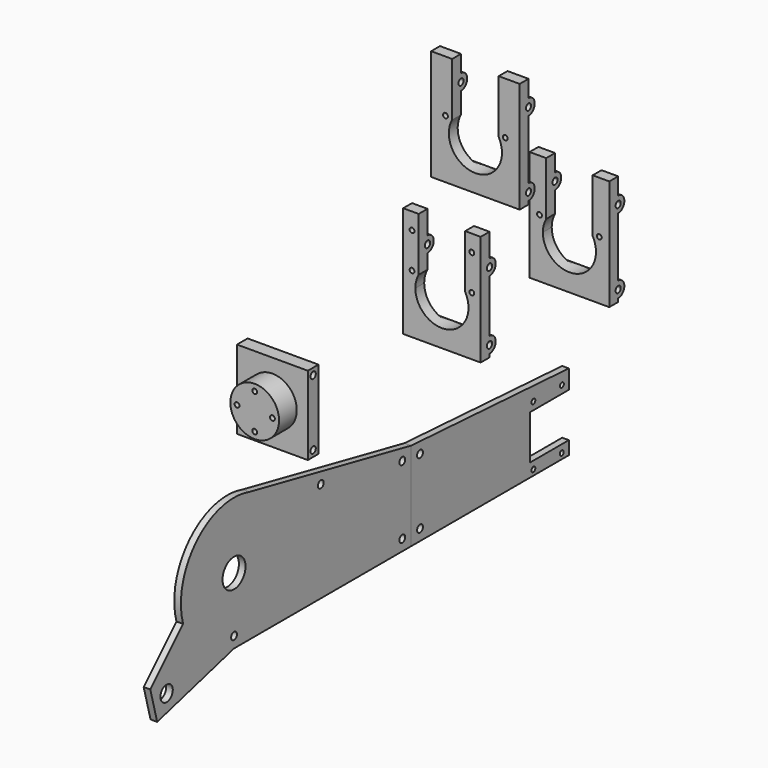
from build123d import *

# Parameters (mm, degrees)
F0_R            = 1.65
F0_R_2          = 1.1
F1_DEPTH        = 3
F2_R            = 3.5
F2_R_2          = 1.65
F2_R_3          = 6.5
F3_DEPTH        = 3
F5_DEPTH        = 35
F7_D            = 2.2
F7_DEPTH        = 12
F7_CBORE_D      = 4
F7_CBORE_DEPTH  = 2
F7_TIP          = 0.6609466809
F6_W            = 21
F6_H            = 10.579
F8_DEPTH        = 25
F8_DEPTH_BACK   = 25
F9_W            = 6
F9_H            = 35.53
F10_DEPTH       = 32
F11_D           = 3
F12_R           = 11
F13_DEPTH       = 16
F14_D           = 2.2
F14_CBORE_D     = 4
F14_CBORE_DEPTH = 13
F16_DEPTH       = 36
F17_W           = 21
F17_H           = 7.7
F18_DEPTH       = 222.8771624415
F18_DEPTH_BACK  = 25
F19_D           = 2.2
F19_DEPTH       = 12
F19_CBORE_D     = 4
F19_CBORE_DEPTH = 2
F19_TIP         = 0.6609466809
F21_DEPTH       = 40
F22_W           = 21
F22_H           = 7.7
F23_DEPTH       = 12.5
F24_D           = 2.2
F24_CBORE_D     = 4
F24_CBORE_DEPTH = 2


# Not quite as in the source:
# - a feature names something its author has since deleted; it is built from what else it names


with BuildPart() as f1:
    # F0 (on Right) → F1 (new body)
    with BuildSketch(Plane.YZ):
        Polygon((134.868821919, -66.8961822494), (45.859821919, -61.4187053263), (45.859821919, -101.4187053263), (134.868821919, -101.4187053263), (134.868821919, -95.4187053263), (112.868821919, -95.4187053263), (112.868821919, -75.4187053263), (134.868821919, -75.4187053263), align=None)
        with Locations((50.859821919, -96.4187053263)):
            Circle(F0_R, mode=Mode.SUBTRACT)
        with Locations((114.868821919, -98.9187053263)):
            Circle(F0_R_2, mode=Mode.SUBTRACT)
        with Locations((130.868821919, -98.9187053263)):
            Circle(F0_R_2, mode=Mode.SUBTRACT)
        with Locations((50.859821919, -66.7358561433)):
            Circle(F0_R, mode=Mode.SUBTRACT)
        with Locations((114.868821919, -71.9187053263)):
            Circle(F0_R_2, mode=Mode.SUBTRACT)
        with Locations((130.9641025662, -71.9187053263)):
            Circle(F0_R_2, mode=Mode.SUBTRACT)
    extrude(amount=F1_DEPTH)


with BuildPart() as f3:
    # F2 (on Right) → F3 (new body)
    with BuildSketch(Plane.YZ):
        with BuildLine():
            Line((45.859821919, -101.4187053263), (45.859821919, -61.4187053263))
            Line((45.859821919, -61.4187053263), (-45.5225354032, -42.683078751))
            ThreePointArc((-45.5225354032, -42.683078751), (-75.3328827835, -50.1850229468), (-82.8923977892, -79.9808231631))
            Line((-82.8923977892, -79.9808231631), (-101.4139502366, -98.5023756104))
            Line((-101.4139502366, -98.5023756104), (-97.5316645601, -112.9912630048))
            Line((-97.5316645601, -112.9912630048), (-54.140178081, -101.4187053263))
            Line((-54.140178081, -101.4187053263), (45.859821919, -101.4187053263))
        make_face()
        with Locations((-92.2261038997, -103.814110163)):
            Circle(F2_R, mode=Mode.SUBTRACT)
        with Locations((-54.140178081, -96.4187053263)):
            Circle(F2_R_2, mode=Mode.SUBTRACT)
        with Locations((40.859821919, -96.4187053263)):
            Circle(F2_R_2, mode=Mode.SUBTRACT)
        with Locations((-54.140178081, -71.4187053263)):
            Circle(F2_R_3, mode=Mode.SUBTRACT)
        with Locations((40.859821919, -65.4975885229)):
            Circle(F2_R_2, mode=Mode.SUBTRACT)
        with Locations((-5.1531680486, -56.0637960173)):
            Circle(F2_R_2, mode=Mode.SUBTRACT)
    extrude(amount=F3_DEPTH)


with BuildPart() as f5:
    # F4 (on Right) → F5 (new body)
    with BuildSketch(Plane.YZ):
        with BuildLine():
            Line((50.0948551297, 21.7378329895), (50.0948551297, 32.3168329895))
            Line((50.0948551297, 32.3168329895), (45.0948551297, 32.3168329895))
            Line((45.0948551297, 32.3168329895), (45.0948551297, -17.6831670105))
            Line((45.0948551297, -17.6831670105), (50.0948551297, -17.6831670105))
            Line((50.0948551297, -17.6831670105), (50.0948551297, -16.1831670105))
            ThreePointArc((50.0948551297, -16.1831670105), (46.5948551297, -12.6831670105), (50.0948551297, -9.1831670105))
            Line((50.0948551297, -9.1831670105), (50.0948551297, 14.7378329895))
            ThreePointArc((50.0948551297, 14.7378329895), (46.5948551297, 18.2378329895), (50.0948551297, 21.7378329895))
        make_face()
        with BuildLine():
            ThreePointArc((53.5948551297, 18.2378329895), (52.5697288639, 20.7127067236), (50.0948551297, 21.7378329895))
            Line((50.0948551297, 21.7378329895), (50.0948551297, 19.7378329895))
            ThreePointArc((50.0948551297, 19.7378329895), (51.1555153015, 19.2984931612), (51.5948551297, 18.2378329895))
            ThreePointArc((51.5948551297, 18.2378329895), (51.1555153015, 17.1771728177), (50.0948551297, 16.7378329895))
            Line((50.0948551297, 16.7378329895), (50.0948551297, 14.7378329895))
            ThreePointArc((50.0948551297, 14.7378329895), (52.5697288639, 15.7629592553), (53.5948551297, 18.2378329895))
        make_face()
        with BuildLine():
            Line((50.0948551297, 19.7378329895), (50.0948551297, 21.7378329895))
            ThreePointArc((50.0948551297, 21.7378329895), (46.5948551297, 18.2378329895), (50.0948551297, 14.7378329895))
            Line((50.0948551297, 14.7378329895), (50.0948551297, 16.7378329895))
            ThreePointArc((50.0948551297, 16.7378329895), (48.5948551297, 18.2378329895), (50.0948551297, 19.7378329895))
        make_face()
        with BuildLine():
            ThreePointArc((53.5948551297, -12.6831670105), (52.5697288639, -10.2082932764), (50.0948551297, -9.1831670105))
            Line((50.0948551297, -9.1831670105), (50.0948551297, -11.1831670105))
            ThreePointArc((50.0948551297, -11.1831670105), (51.1555153015, -11.6225068388), (51.5948551297, -12.6831670105))
            ThreePointArc((51.5948551297, -12.6831670105), (51.1555153015, -13.7438271823), (50.0948551297, -14.1831670105))
            Line((50.0948551297, -14.1831670105), (50.0948551297, -16.1831670105))
            ThreePointArc((50.0948551297, -16.1831670105), (52.5697288639, -15.1580407447), (53.5948551297, -12.6831670105))
        make_face()
        with BuildLine():
            Line((50.0948551297, -11.1831670105), (50.0948551297, -9.1831670105))
            ThreePointArc((50.0948551297, -9.1831670105), (46.5948551297, -12.6831670105), (50.0948551297, -16.1831670105))
            Line((50.0948551297, -16.1831670105), (50.0948551297, -14.1831670105))
            ThreePointArc((50.0948551297, -14.1831670105), (48.5948551297, -12.6831670105), (50.0948551297, -11.1831670105))
        make_face()
    extrude(amount=F5_DEPTH)

    # F7
    with Locations(Plane(origin=(0, 50.0948551297, 0), x_dir=(-1, 0, 0), z_dir=(0, 1, 0))):
        with Locations((-4, 24.8168329895), (-4, 8.8168329895), (-31, 24.8168329895), (-31, 8.8168329895)):
            CounterBoreHole(F7_D / 2, F7_CBORE_D / 2, F7_CBORE_DEPTH, depth=F7_DEPTH)
            with Locations((0, 0, -(F7_DEPTH + F7_TIP / 2))):  # 118° drill point
                Cone(0, F7_D / 2, F7_TIP, mode=Mode.SUBTRACT)

    # F6 (on face) → F8 (cut, two sides)
    with BuildSketch(Plane(origin=(0, 50.0948551297, 0), x_dir=(-1, 0, 0), z_dir=(0, 1, 0))) as f8_sk:
        with BuildLine():
            ThreePointArc((-28, 8.1263080088), (-20.5, -9.3021170492), (-5.5, 2.3168329895))
            ThreePointArc((-5.5, 2.3168329895), (-5.8810499614, 5.3168329895), (-7, 8.1263080088))
            ThreePointArc((-7, 8.1263080088), (-17.5, 14.3168329895), (-28, 8.1263080088))
        make_face()
        with BuildLine():
            ThreePointArc((-28, 8.1263080088), (-17.5, 14.3168329895), (-7, 8.1263080088))
            Line((-7, 8.1263080088), (-7, 21.7378329895))
            Line((-7, 21.7378329895), (-28, 21.7378329895))
            Line((-28, 21.7378329895), (-28, 8.1263080088))
        make_face()
        with Locations((-17.5, 27.0273329895)):
            Rectangle(F6_W, F6_H)
    extrude(amount=-F8_DEPTH, mode=Mode.SUBTRACT)
    extrude(f8_sk.sketch, amount=F8_DEPTH_BACK, mode=Mode.SUBTRACT)


with BuildPart() as f10:
    # F9 (on Right) → F10 (new body)
    with BuildSketch(Plane.YZ):
        with Locations((-45.7222016811, -1.5251142904)):
            Rectangle(F9_W, F9_H)
    extrude(amount=F10_DEPTH)

    # F11 (through all)
    with Locations(Plane(origin=(0, 0, 0), x_dir=(0, 1, 0), z_dir=(-1, 0, 0))):
        with Locations((-45.7222016811, -13.2398857096), (-45.7222016811, 16.4431142904)):
            Hole(F11_D / 2)

    # F12 (on face) → F13 (join)
    with BuildSketch(Plane(origin=(0, -42.7222016811, 0), x_dir=(-1, 0, 0), z_dir=(0, 1, 0))):
        with Locations((-16, -1.0909485864)):
            Circle(F12_R)
    extrude(amount=-F13_DEPTH)

    # F14 (through all)
    with Locations(Plane(origin=(0, -42.7222016811, 0), x_dir=(-1, 0, 0), z_dir=(0, 1, 0))):
        with Locations((-16, 6.9090514136), (-8, -1.0909485864), (-16, -9.0909485864), (-24, -1.0909485864)):
            CounterBoreHole(F14_D / 2, F14_CBORE_D / 2, F14_CBORE_DEPTH)


with BuildPart() as f16:
    # F15 (on Right) → F16 (new body)
    with BuildSketch(Plane.YZ):
        with BuildLine():
            Line((121.4622122049, 17.9643252028), (121.4622122049, 25.6643252028))
            Line((121.4622122049, 25.6643252028), (116.4622122049, 25.6643252028))
            Line((116.4622122049, 25.6643252028), (116.4622122049, -24.3356747972))
            Line((116.4622122049, -24.3356747972), (121.4622122049, -24.3356747972))
            Line((121.4622122049, -24.3356747972), (121.4622122049, -22.8356747972))
            ThreePointArc((121.4622122049, -22.8356747972), (117.9622122049, -19.3356747972), (121.4622122049, -15.8356747972))
            Line((121.4622122049, -15.8356747972), (121.4622122049, 10.9643252028))
            ThreePointArc((121.4622122049, 10.9643252028), (117.9622122049, 14.4643252028), (121.4622122049, 17.9643252028))
        make_face()
        with BuildLine():
            ThreePointArc((124.9622122049, 14.4643252028), (123.9370859391, 16.939198937), (121.4622122049, 17.9643252028))
            Line((121.4622122049, 17.9643252028), (121.4622122049, 15.9143252028))
            ThreePointArc((121.4622122049, 15.9143252028), (122.4875170377, 15.4896300356), (122.9122122049, 14.4643252028))
            ThreePointArc((122.9122122049, 14.4643252028), (122.4875170377, 13.4390203701), (121.4622122049, 13.0143252028))
            Line((121.4622122049, 13.0143252028), (121.4622122049, 10.9643252028))
            ThreePointArc((121.4622122049, 10.9643252028), (123.9370859391, 11.9894514687), (124.9622122049, 14.4643252028))
        make_face()
        with BuildLine():
            Line((121.4622122049, 15.9143252028), (121.4622122049, 17.9643252028))
            ThreePointArc((121.4622122049, 17.9643252028), (117.9622122049, 14.4643252028), (121.4622122049, 10.9643252028))
            Line((121.4622122049, 10.9643252028), (121.4622122049, 13.0143252028))
            ThreePointArc((121.4622122049, 13.0143252028), (120.0122122049, 14.4643252028), (121.4622122049, 15.9143252028))
        make_face()
        with BuildLine():
            ThreePointArc((124.9622122049, -19.3356747972), (123.9370859391, -16.860801063), (121.4622122049, -15.8356747972))
            Line((121.4622122049, -15.8356747972), (121.4622122049, -17.8856747972))
            ThreePointArc((121.4622122049, -17.8856747972), (122.4875170377, -18.3103699644), (122.9122122049, -19.3356747972))
            ThreePointArc((122.9122122049, -19.3356747972), (122.4875170377, -20.3609796299), (121.4622122049, -20.7856747972))
            Line((121.4622122049, -20.7856747972), (121.4622122049, -22.8356747972))
            ThreePointArc((121.4622122049, -22.8356747972), (123.9370859391, -21.8105485313), (124.9622122049, -19.3356747972))
        make_face()
        with BuildLine():
            Line((121.4622122049, -17.8856747972), (121.4622122049, -15.8356747972))
            ThreePointArc((121.4622122049, -15.8356747972), (117.9622122049, -19.3356747972), (121.4622122049, -22.8356747972))
            Line((121.4622122049, -22.8356747972), (121.4622122049, -20.7856747972))
            ThreePointArc((121.4622122049, -20.7856747972), (120.0122122049, -19.3356747972), (121.4622122049, -17.8856747972))
        make_face()
    extrude(amount=F16_DEPTH)

    # F17 (on face) → F18 (cut, two sides)
    with BuildSketch(Plane(origin=(0, 121.4622122049, 0), x_dir=(-1, 0, 0), z_dir=(0, 1, 0))) as f18_sk:
        with BuildLine():
            ThreePointArc((-28.5, 1.4738002221), (-21, -15.9546248358), (-6, -4.3356747972))
            ThreePointArc((-6, -4.3356747972), (-6.3810499614, -1.3356747972), (-7.5, 1.4738002221))
            ThreePointArc((-7.5, 1.4738002221), (-18, 7.6643252028), (-28.5, 1.4738002221))
        make_face()
        with Locations((-18, 21.8143252028)):
            Rectangle(F17_W, F17_H)
        with BuildLine():
            ThreePointArc((-28.5, 1.4738002221), (-18, 7.6643252028), (-7.5, 1.4738002221))
            Line((-7.5, 1.4738002221), (-7.5, 17.9643252028))
            Line((-7.5, 17.9643252028), (-28.5, 17.9643252028))
            Line((-28.5, 17.9643252028), (-28.5, 1.4738002221))
        make_face()
    extrude(amount=-F18_DEPTH, mode=Mode.SUBTRACT)
    extrude(f18_sk.sketch, amount=F18_DEPTH_BACK, mode=Mode.SUBTRACT)

    # F19
    with Locations(Plane(origin=(0, 121.4622122049, 0), x_dir=(-1, 0, 0), z_dir=(0, 1, 0))):
        with Locations((-31.5, 2.1643252028), (-4.5, 2.1643252028)):
            CounterBoreHole(F19_D / 2, F19_CBORE_D / 2, F19_CBORE_DEPTH, depth=F19_DEPTH)
            with Locations((0, 0, -(F19_DEPTH + F19_TIP / 2))):  # 118° drill point
                Cone(0, F19_D / 2, F19_TIP, mode=Mode.SUBTRACT)


with BuildPart() as f21:
    # F20 (on Right) → F21 (new body)
    with BuildSketch(Plane.YZ):
        with BuildLine():
            Line((65.8788916469, 80.6316277573), (65.8788916469, 88.3316277573))
            Line((65.8788916469, 88.3316277573), (60.8788916469, 88.3316277573))
            Line((60.8788916469, 88.3316277573), (60.8788916469, 38.3316277573))
            Line((60.8788916469, 38.3316277573), (65.8788916469, 38.3316277573))
            Line((65.8788916469, 38.3316277573), (65.8788916469, 39.8316277573))
            ThreePointArc((65.8788916469, 39.8316277573), (62.3788916469, 43.3316277573), (65.8788916469, 46.8316277573))
            Line((65.8788916469, 46.8316277573), (65.8788916469, 73.6316277573))
            ThreePointArc((65.8788916469, 73.6316277573), (62.3788916469, 77.1316277573), (65.8788916469, 80.6316277573))
        make_face()
        with BuildLine():
            ThreePointArc((69.3788916469, 77.1316277573), (68.353765381, 79.6065014915), (65.8788916469, 80.6316277573))
            Line((65.8788916469, 80.6316277573), (65.8788916469, 78.5816277573))
            ThreePointArc((65.8788916469, 78.5816277573), (66.9041964796, 78.15693259), (67.3288916469, 77.1316277573))
            ThreePointArc((67.3288916469, 77.1316277573), (66.9041964796, 76.1063229246), (65.8788916469, 75.6816277573))
            Line((65.8788916469, 75.6816277573), (65.8788916469, 73.6316277573))
            ThreePointArc((65.8788916469, 73.6316277573), (68.353765381, 74.6567540232), (69.3788916469, 77.1316277573))
        make_face()
        with BuildLine():
            Line((65.8788916469, 78.5816277573), (65.8788916469, 80.6316277573))
            ThreePointArc((65.8788916469, 80.6316277573), (62.3788916469, 77.1316277573), (65.8788916469, 73.6316277573))
            Line((65.8788916469, 73.6316277573), (65.8788916469, 75.6816277573))
            ThreePointArc((65.8788916469, 75.6816277573), (64.4288916469, 77.1316277573), (65.8788916469, 78.5816277573))
        make_face()
        with BuildLine():
            ThreePointArc((69.3788916469, 43.3316277573), (68.353765381, 45.8065014915), (65.8788916469, 46.8316277573))
            Line((65.8788916469, 46.8316277573), (65.8788916469, 44.7816277573))
            ThreePointArc((65.8788916469, 44.7816277573), (66.9041964796, 44.35693259), (67.3288916469, 43.3316277573))
            ThreePointArc((67.3288916469, 43.3316277573), (66.9041964796, 42.3063229246), (65.8788916469, 41.8816277573))
            Line((65.8788916469, 41.8816277573), (65.8788916469, 39.8316277573))
            ThreePointArc((65.8788916469, 39.8316277573), (68.353765381, 40.8567540232), (69.3788916469, 43.3316277573))
        make_face()
        with BuildLine():
            Line((65.8788916469, 44.7816277573), (65.8788916469, 46.8316277573))
            ThreePointArc((65.8788916469, 46.8316277573), (62.3788916469, 43.3316277573), (65.8788916469, 39.8316277573))
            Line((65.8788916469, 39.8316277573), (65.8788916469, 41.8816277573))
            ThreePointArc((65.8788916469, 41.8816277573), (64.4288916469, 43.3316277573), (65.8788916469, 44.7816277573))
        make_face()
    extrude(amount=F21_DEPTH)

    # F22 (on face) → F23 (cut, symmetric)
    with BuildSketch(Plane(origin=(0, 65.8788916469, 0), x_dir=(-1, 0, 0), z_dir=(0, 1, 0))):
        with Locations((-20, 84.4816277573)):
            Rectangle(F22_W, F22_H)
        with BuildLine():
            ThreePointArc((-30.5, 64.1411027766), (-23, 46.7126777187), (-8, 58.3316277573))
            ThreePointArc((-8, 58.3316277573), (-8.3810499614, 61.3316277573), (-9.5, 64.1411027766))
            ThreePointArc((-9.5, 64.1411027766), (-20, 70.3316277573), (-30.5, 64.1411027766))
        make_face()
        with BuildLine():
            ThreePointArc((-30.5, 64.1411027766), (-20, 70.3316277573), (-9.5, 64.1411027766))
            Line((-9.5, 64.1411027766), (-9.5, 80.6316277573))
            Line((-9.5, 80.6316277573), (-30.5, 80.6316277573))
            Line((-30.5, 80.6316277573), (-30.5, 64.1411027766))
        make_face()
    extrude(amount=F23_DEPTH, both=True, mode=Mode.SUBTRACT)

    # F24 (through all)
    with Locations(Plane(origin=(0, 65.8788916469, 0), x_dir=(-1, 0, 0), z_dir=(0, 1, 0))):
        with Locations((-33.5, 64.8316277573), (-6.5, 64.8316277573)):
            CounterBoreHole(F24_D / 2, F24_CBORE_D / 2, F24_CBORE_DEPTH)


solid = Compound([f1.part, f3.part, f5.part, f10.part, f16.part, f21.part])
